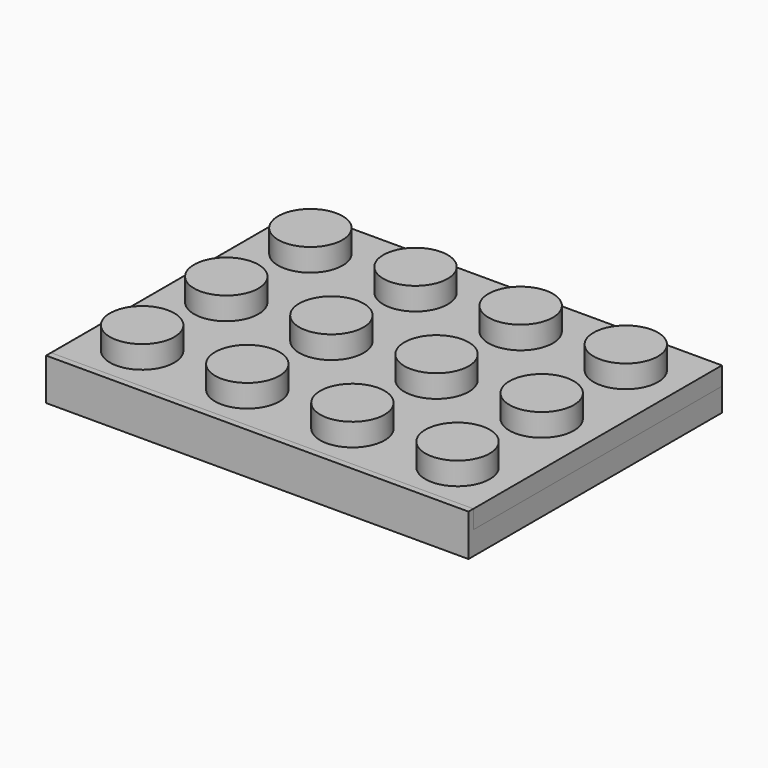
from build123d import *

# Parameters (mm, degrees)
F0_W     = 32.14
F0_H     = 3.18
F1_DEPTH = 24.1
F2_R     = 2.45
F3_DEPTH = 1.72
F4_W     = 29.08
F4_H     = 21.04
F5_DEPTH = 3.5
F6_W     = 32.0825448725
F6_H     = 23.6320719123
F7_DEPTH = 1.4
F8_W     = 1
F8_H     = 1.98
F8_W_2   = 1.152671826
F8_H_2   = 0.75
F8_W_3   = 0.887328174
F8_H_3   = 7.2
F8_H_4   = 7.59
F8_W_4   = 1.223020737
F8_W_5   = 0.816979263
F8_R     = 1.54
F8_R_2   = 0.71
F8_R_3   = 3.25
F8_R_4   = 2.43
F9_DEPTH = 3


with BuildPart() as f1:
    # F0 (on Front) → F1 (new body)
    with BuildSketch(Plane.XZ):
        with Locations((13.9988805842, -1.59)):
            Rectangle(F0_W, F0_H)
    extrude(amount=F1_DEPTH)

    # F4 (on Top) → F5 (cut)
    with BuildSketch(Plane.XY):
        with Locations((13.9988805842, -12.05)):
            Rectangle(F4_W, F4_H)
    extrude(amount=-F5_DEPTH, mode=Mode.SUBTRACT)


with BuildPart() as f3:
    # F2 (on Top) → F3 (new body)
    with BuildSketch(Plane.XY):
        with Locations((1.9988805842, -4.05)):
            Circle(F2_R)
    extrude(amount=F3_DEPTH)


with BuildPart() as f3b:
    # F2 (on Top) → F3, piece 2 (new body)
    with BuildSketch(Plane.XY):
        with Locations((9.9988805842, -4.05)):
            Circle(F2_R)
    extrude(amount=F3_DEPTH)


with BuildPart() as f3c:
    # F2 (on Top) → F3, piece 3 (new body)
    with BuildSketch(Plane.XY):
        with Locations((17.9988805842, -4.05)):
            Circle(F2_R)
    extrude(amount=F3_DEPTH)


with BuildPart() as f3d:
    # F2 (on Top) → F3, piece 4 (new body)
    with BuildSketch(Plane.XY):
        with Locations((25.9988805842, -4.05)):
            Circle(F2_R)
    extrude(amount=F3_DEPTH)


with BuildPart() as f3e:
    # F2 (on Top) → F3, piece 5 (new body)
    with BuildSketch(Plane.XY):
        with Locations((25.9988805842, -12.05)):
            Circle(F2_R)
    extrude(amount=F3_DEPTH)


with BuildPart() as f3f:
    # F2 (on Top) → F3, piece 6 (new body)
    with BuildSketch(Plane.XY):
        with Locations((25.9988805842, -20.05)):
            Circle(F2_R)
    extrude(amount=F3_DEPTH)


with BuildPart() as f3g:
    # F2 (on Top) → F3, piece 7 (new body)
    with BuildSketch(Plane.XY):
        with Locations((17.9988805842, -12.05)):
            Circle(F2_R)
    extrude(amount=F3_DEPTH)


with BuildPart() as f3h:
    # F2 (on Top) → F3, piece 8 (new body)
    with BuildSketch(Plane.XY):
        with Locations((17.9988805842, -20.05)):
            Circle(F2_R)
    extrude(amount=F3_DEPTH)


with BuildPart() as f3i:
    # F2 (on Top) → F3, piece 9 (new body)
    with BuildSketch(Plane.XY):
        with Locations((9.9988805842, -12.05)):
            Circle(F2_R)
    extrude(amount=F3_DEPTH)


with BuildPart() as f3j:
    # F2 (on Top) → F3, piece 10 (new body)
    with BuildSketch(Plane.XY):
        with Locations((9.9988805842, -20.05)):
            Circle(F2_R)
    extrude(amount=F3_DEPTH)


with BuildPart() as f3k:
    # F2 (on Top) → F3, piece 11 (new body)
    with BuildSketch(Plane.XY):
        with Locations((1.9988805842, -12.05)):
            Circle(F2_R)
    extrude(amount=F3_DEPTH)


with BuildPart() as f3l:
    # F2 (on Top) → F3, piece 12 (new body)
    with BuildSketch(Plane.XY):
        with Locations((1.9988805842, -20.05)):
            Circle(F2_R)
    extrude(amount=F3_DEPTH)


with BuildPart() as f7:
    # F6 (on Top) → F7 (new body)
    with BuildSketch(Plane.XY):
        with Locations((14.0309714479, -11.8160359561)):
            Rectangle(F6_W, F6_H)
    extrude(amount=-F7_DEPTH)

    # F8 (on Top) → F9 (join)
    with BuildSketch(Plane.XY):
        with Locations((5.7688805842, -21.54)):
            Rectangle(F8_W, F8_H)
        with Locations((4.6925446712, -20.175)):
            Rectangle(F8_W_2, F8_H_2)
        with Locations((5.7688805842, -20.175)):
            Rectangle(F8_W, F8_H_2)
        with Locations((6.7125446712, -20.175)):
            Rectangle(F8_W_3, F8_H_2)
        with Locations((5.7688805842, -16.2)):
            Rectangle(F8_W, F8_H_3)
        with Locations((4.6925446712, -12.225)):
            Rectangle(F8_W_2, F8_H_2)
        with Locations((5.7688805842, -12.225)):
            Rectangle(F8_W, F8_H_2)
        with Locations((6.7125446712, -12.225)):
            Rectangle(F8_W_3, F8_H_2)
        with Locations((5.7688805842, -8.055)):
            Rectangle(F8_W, F8_H_4)
        with Locations((4.6925446712, -3.885)):
            Rectangle(F8_W_2, F8_H_2)
        with Locations((5.7688805842, -3.885)):
            Rectangle(F8_W, F8_H_2)
        with Locations((6.7125446712, -3.885)):
            Rectangle(F8_W_3, F8_H_2)
        with Locations((5.7688805842, -2.52)):
            Rectangle(F8_W, F8_H)
        with Locations((22.2288805842, -21.54)):
            Rectangle(F8_W, F8_H)
        with Locations((21.1173702157, -20.175)):
            Rectangle(F8_W_4, F8_H_2)
        with Locations((22.2288805842, -20.175)):
            Rectangle(F8_W, F8_H_2)
        with Locations((23.1373702157, -20.175)):
            Rectangle(F8_W_5, F8_H_2)
        with Locations((22.2288805842, -16.2)):
            Rectangle(F8_W, F8_H_3)
        with Locations((21.1173702157, -12.225)):
            Rectangle(F8_W_4, F8_H_2)
        with Locations((22.2288805842, -12.225)):
            Rectangle(F8_W, F8_H_2)
        with Locations((23.1373702157, -12.225)):
            Rectangle(F8_W_5, F8_H_2)
        with Locations((22.2288805842, -8.055)):
            Rectangle(F8_W, F8_H_4)
        with Locations((21.1173702157, -3.885)):
            Rectangle(F8_W_4, F8_H_2)
        with Locations((22.2288805842, -3.885)):
            Rectangle(F8_W, F8_H_2)
        with Locations((23.1373702157, -3.885)):
            Rectangle(F8_W_5, F8_H_2)
        with Locations((22.2288805842, -2.52)):
            Rectangle(F8_W, F8_H)
        with Locations((1.8888805842, -7.792100538)):
            Circle(F8_R)
        with Locations((1.8888805842, -7.792100538)):
            Circle(F8_R_2, mode=Mode.SUBTRACT)
        with Locations((1.8888805842, -15.772100538)):
            Circle(F8_R)
        with Locations((1.8888805842, -15.772100538)):
            Circle(F8_R_2, mode=Mode.SUBTRACT)
        with Locations((25.7731880212, -15.772100538)):
            Circle(F8_R)
        with Locations((25.7731880212, -15.772100538)):
            Circle(F8_R_2, mode=Mode.SUBTRACT)
        with Locations((25.7731880212, -7.792100538)):
            Circle(F8_R)
        with Locations((25.7731880212, -7.792100538)):
            Circle(F8_R_2, mode=Mode.SUBTRACT)
        with Locations((13.8310343027, -15.772100538)):
            Circle(F8_R_3)
        with Locations((13.8310343027, -15.772100538)):
            Circle(F8_R_4, mode=Mode.SUBTRACT)
        with Locations((13.8310343027, -7.792100538)):
            Circle(F8_R_3)
        with Locations((13.8310343027, -7.792100538)):
            Circle(F8_R_4, mode=Mode.SUBTRACT)
    extrude(amount=-F9_DEPTH)


solid = Compound([f1.part, f3.part, f3b.part, f3c.part, f3d.part, f3e.part, f3f.part, f3g.part, f3h.part, f3i.part, f3j.part, f3k.part, f3l.part, f7.part])
